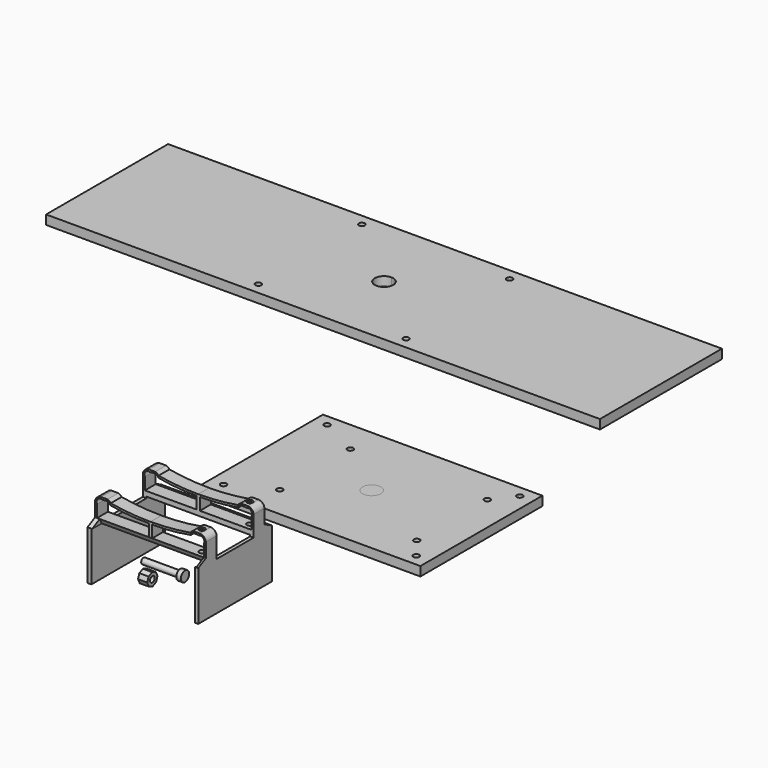
from build123d import *

# Parameters (mm, degrees)
F1_DEPTH  = 60
F3_DEPTH  = 44.8691186885
F5_DEPTH  = 50.001
F7_DEPTH  = 25
F0_R      = 1.6
F8_DEPTH  = 20
F9_R      = 2.7879573669
F9_R_2    = 1.6
F10_DEPTH = 2.5
F11_DEPTH = 5
F12_R     = 1.6
F13_DEPTH = 25
F15_R     = 1.6
F16_DEPTH = 25
F14_W     = 84.7538411142
F14_H     = 58.092317279
F14_R     = 1.6
F17_DEPTH = 5
F14_W_2   = 118.871630811
F14_H_2   = 82.6016969972
F18_DEPTH = 5
F19_R     = 5
F20_DEPTH = 25
F21_DEPTH = 5


# Not quite as in the source:
# - a feature names something its author has since deleted; it is built from what else it names


with BuildPart() as f1:
    # F0 (on Right) → F1 (new body)
    with BuildSketch(Plane.YZ):
        Polygon((-12.5, 20), (-19.8681186885, 20), (-19.8681186885, 9.2717893422), (-25, 6.6227070056), (-25, -20), (25, -20), (25, 6.6227070056), (19.8681186885, 9.2717893422), (19.8681186885, 20), (12.5, 20), (12.5, 5.9002293274), (0, 5.9002293274), (-12.5, 5.9002293274), align=None)
    extrude(amount=-F1_DEPTH)

    # F2 (on face) → F3 (cut, through all)
    with BuildSketch(Plane.XZ.offset(19.8681186885)):
        with BuildLine():
            ThreePointArc((-60, 16.9909157804), (-58.932532239, 19.0893193514), (-56.7614850899, 20))
            Line((-56.7614850899, 20), (-60, 20))
            Line((-60, 20), (-60, 16.9909157804))
        make_face()
        with BuildLine():
            Line((0, 20), (-3.2385149101, 20))
            ThreePointArc((-3.2385149101, 20), (-1.067467761, 19.0893193514), (0, 16.9909157804))
            Line((0, 16.9909157804), (0, 20))
        make_face()
        with BuildLine():
            Line((-30, 20), (-53.2782711089, 20))
            ThreePointArc((-53.2782711089, 20), (-52.2794249104, 19.5204218101), (-51.5175877356, 18.7158765425))
            ThreePointArc((-51.5175877356, 18.7158765425), (-40.7972581254, 17.3508340995), (-30, 16.894736748))
            Line((-30, 16.894736748), (-30, 20))
        make_face()
        with BuildLine():
            Line((-6.7217288911, 20), (-30, 20))
            Line((-30, 20), (-30, 16.894736748))
            ThreePointArc((-30, 16.894736748), (-19.2027418746, 17.3508340995), (-8.4824122644, 18.7158765425))
            ThreePointArc((-8.4824122644, 18.7158765425), (-7.7205750896, 19.5204218101), (-6.7217288911, 20))
        make_face()
        with BuildLine():
            Line((-58.9228533208, 15.9691069275), (-58.9228533208, 9.2717893422))
            Line((-58.9228533208, 9.2717893422), (-30.8992173523, 9.2717893422))
            Line((-30.8992173523, 9.2717893422), (-30.8992173523, 15.8769246191))
            ThreePointArc((-30.8992173523, 15.8769246191), (-41.4569313238, 16.2418451853), (-51.9169420004, 17.7205838263))
            ThreePointArc((-51.9169420004, 17.7205838263), (-52.2168663975, 18.8034052316), (-53.2996878028, 19.1033296287))
            Line((-53.2996878028, 19.1033296287), (-56.4339123666, 18.9189631492))
            ThreePointArc((-56.4339123666, 18.9189631492), (-58.697924797, 18.3042734809), (-58.9228533208, 15.9691069275))
        make_face()
        with BuildLine():
            Line((-29.1007826477, 15.8769246191), (-29.1007826477, 9.2717893422))
            Line((-29.1007826477, 9.2717893422), (-1.0771466792, 9.2717893422))
            Line((-1.0771466792, 9.2717893422), (-1.0771466792, 15.9691069275))
            ThreePointArc((-1.0771466792, 15.9691069275), (-1.302075203, 18.3042734809), (-3.5660876334, 18.9189631492))
            Line((-3.5660876334, 18.9189631492), (-6.7003121972, 19.1033296287))
            ThreePointArc((-6.7003121972, 19.1033296287), (-7.7831336025, 18.8034052316), (-8.0830579996, 17.7205838263))
            ThreePointArc((-8.0830579996, 17.7205838263), (-18.5430686762, 16.2418451853), (-29.1007826477, 15.8769246191))
        make_face()
    extrude(amount=-F3_DEPTH, mode=Mode.SUBTRACT)

    # F4 (on face) → F5 (cut, through all)
    with BuildSketch(Plane.XZ.offset(25)):
        Polygon((-57.9314492643, 5.0185960717), (-57.9314492643, -20), (-1.8841834972, -20), (-1.8841834972, 5.0185960717), (-1.8841834972, 6.6227070056), (-57.9314492643, 6.6227070056), align=None)
    extrude(amount=-F5_DEPTH, mode=Mode.SUBTRACT)

    # F6 (on face) → F7 (cut)
    with BuildSketch(Plane(origin=(0, -7.959357176, 15.41910411), x_dir=(1, 0, 0), z_dir=(0, -0.4586934268, 0.8885945871))):
        Polygon((-57.4829429388, -13.4017938954), (-57.4829429388, -19.1770725053), (-1.8841834972, -19.1770725053), (-1.0771466792, -19.1770725053), (-1.0771466792, -13.4017938954), (-29.1007826477, -13.4017938954), (-30.8992173523, -13.4017938954), align=None)
    extrude(amount=-F7_DEPTH, mode=Mode.SUBTRACT)

    # F12 (on face) → F13 (cut)
    with BuildSketch(Plane.XY.offset(20)):
        with Locations((-4.9801219006, -16.1840593442)):
            Circle(F12_R)
    extrude(amount=-F13_DEPTH, mode=Mode.SUBTRACT)

    # F15 (on face) → F16 (cut)
    with BuildSketch(Plane.XY.offset(20)):
        with Locations((-4.9801219006, 16.1840593442)):
            Circle(F15_R)
    extrude(amount=-F16_DEPTH, mode=Mode.SUBTRACT)


with BuildPart() as f8:
    # F0 (on Right) → F8 (new body)
    with BuildSketch(Plane.YZ):
        with Locations((-62.0705150068, 25.1176990569)):
            Circle(F0_R)
    extrude(amount=F8_DEPTH)

    # F9 (on face) → F10 (join)
    with BuildSketch(Plane.YZ.offset(20)):
        with Locations((-62.0705150068, 25.1176990569)):
            Circle(F9_R)
        with Locations((-62.0705150068, 25.1176990569)):
            Circle(F9_R_2, mode=Mode.SUBTRACT)
        with Locations((-62.0705150068, 25.1176990569)):
            Circle(F9_R_2)
    extrude(amount=F10_DEPTH)


with BuildPart() as f11:
    # F0 (on Right) → F11 (new body)
    with BuildSketch(Plane.YZ):
        Polygon((-64.8864083534, 20.4282177635), (-65.7864786143, 17.9275685899), (-64.6546984114, 15.5228968168), (-62.1540492378, 14.6228265559), (-59.7493774647, 15.7546067588), (-58.8493072038, 18.2552559324), (-59.9810874067, 20.6599277054), (-62.4817365803, 21.5599979664), align=None)
        with Locations((-62.317892909, 18.0914122611)):
            Circle(F0_R, mode=Mode.SUBTRACT)
    extrude(amount=F11_DEPTH)


with BuildPart() as f17:
    # F14 (on Top) → F17 (new body)
    with BuildSketch(Plane.XY):
        with Locations((17.2538864457, 78.9265636351)):
            Rectangle(F14_W, F14_H)
        with Locations((-19.8619253933, 55.0478957593)):
            Circle(F14_R, mode=Mode.SUBTRACT)
        with Locations((-5.2461135543, 62.7415636351)):
            Circle(F14_R, mode=Mode.SUBTRACT)
        with Locations((39.7538864457, 62.7415636351)):
            Circle(F14_R, mode=Mode.SUBTRACT)
        with Locations((54.3696982848, 55.0478957593)):
            Circle(F14_R, mode=Mode.SUBTRACT)
        with Locations((-5.2461135543, 95.1115636351)):
            Circle(F14_R, mode=Mode.SUBTRACT)
        with Locations((39.7538864457, 95.1115636351)):
            Circle(F14_R, mode=Mode.SUBTRACT)
        with Locations((-19.8619253933, 102.8052315109)):
            Circle(F14_R, mode=Mode.SUBTRACT)
        with Locations((54.3696982848, 102.8052315109)):
            Circle(F14_R, mode=Mode.SUBTRACT)
    extrude(amount=F17_DEPTH)


with BuildPart() as f18:
    # F14 (on Top) → F18 (new body)
    with BuildSketch(Plane.XY):
        with Locations((10.8154333714, 78.9265636351)):
            Rectangle(F14_W_2, F14_H_2)
        with Locations((-41.4045543306, 43.8686199486)):
            Circle(F14_R, mode=Mode.SUBTRACT)
        with Locations((63.0354210734, 43.8686199486)):
            Circle(F14_R, mode=Mode.SUBTRACT)
        with Locations((17.2538864457, 78.9265636351)):
            Rectangle(F14_W, F14_H, mode=Mode.SUBTRACT)
        with Locations((-41.4045543306, 113.9845073217)):
            Circle(F14_R, mode=Mode.SUBTRACT)
        with Locations((63.0354210734, 113.9845073217)):
            Circle(F14_R, mode=Mode.SUBTRACT)
        with Locations((17.2538864457, 78.9265636351)):
            Rectangle(F14_W, F14_H)
        with Locations((-19.8619253933, 55.0478957593)):
            Circle(F14_R, mode=Mode.SUBTRACT)
        with Locations((-5.2461135543, 62.7415636351)):
            Circle(F14_R, mode=Mode.SUBTRACT)
        with Locations((39.7538864457, 62.7415636351)):
            Circle(F14_R, mode=Mode.SUBTRACT)
        with Locations((54.3696982848, 55.0478957593)):
            Circle(F14_R, mode=Mode.SUBTRACT)
        with Locations((-5.2461135543, 95.1115636351)):
            Circle(F14_R, mode=Mode.SUBTRACT)
        with Locations((39.7538864457, 95.1115636351)):
            Circle(F14_R, mode=Mode.SUBTRACT)
        with Locations((-19.8619253933, 102.8052315109)):
            Circle(F14_R, mode=Mode.SUBTRACT)
        with Locations((54.3696982848, 102.8052315109)):
            Circle(F14_R, mode=Mode.SUBTRACT)
        with Locations((-5.2461135543, 62.7415636351)):
            Circle(F14_R)
        with Locations((-5.2461135543, 95.1115636351)):
            Circle(F14_R)
        with Locations((39.7538864457, 95.1115636351)):
            Circle(F14_R)
        with Locations((39.7538864457, 62.7415636351)):
            Circle(F14_R)
    extrude(amount=F18_DEPTH)

    # F19 (on face) → F20 (cut)
    with BuildSketch(Plane(origin=(0, 0, 0), x_dir=(1, 0, 0), z_dir=(0, 0, -1))):
        with Locations((10.8154333714, -78.9265636351)):
            Circle(F19_R)
    extrude(amount=-F20_DEPTH, mode=Mode.SUBTRACT)


with BuildPart() as f21:
    # F14 (on Top) → F21 (new body)
    with BuildSketch(Plane.XY):
        with BuildLine():
            Line((-104.5947372913, 236.5341544628), (-104.5947372913, 272.8341544628))
            Line((-104.5947372913, 272.8341544628), (-254.6290494502, 272.8341544628))
            Line((-254.6290494502, 272.8341544628), (-254.6290494502, 190.2341544628))
            Line((-254.6290494502, 190.2341544628), (-104.5947372913, 190.2341544628))
            Line((-104.5947372913, 190.2341544628), (-104.5947372913, 226.5341544628))
            ThreePointArc((-104.5947372913, 226.5341544628), (-109.5947372913, 231.5341544628), (-104.5947372913, 236.5341544628))
        make_face()
        with Locations((-144.5947372913, 196.4770544628)):
            Circle(F14_R, mode=Mode.SUBTRACT)
        with Locations((-144.5947372913, 266.5912544628)):
            Circle(F14_R, mode=Mode.SUBTRACT)
        with BuildLine():
            Line((45.4395748675, 190.2341544628), (45.4395748675, 272.8341544628))
            Line((45.4395748675, 272.8341544628), (-104.5947372913, 272.8341544628))
            Line((-104.5947372913, 272.8341544628), (-104.5947372913, 236.5341544628))
            ThreePointArc((-104.5947372913, 236.5341544628), (-101.0592033854, 235.0696883687), (-99.5947372913, 231.5341544628))
            ThreePointArc((-99.5947372913, 231.5341544628), (-101.0592033854, 227.9986205569), (-104.5947372913, 226.5341544628))
            Line((-104.5947372913, 226.5341544628), (-104.5947372913, 190.2341544628))
            Line((-104.5947372913, 190.2341544628), (45.4395748675, 190.2341544628))
        make_face()
        with Locations((-64.5947372913, 196.4770544628)):
            Circle(F14_R, mode=Mode.SUBTRACT)
        with Locations((-64.5947372913, 266.5912544628)):
            Circle(F14_R, mode=Mode.SUBTRACT)
    extrude(amount=F21_DEPTH)


solid = Compound([f1.part, f8.part, f11.part, f17.part, f18.part, f21.part])
